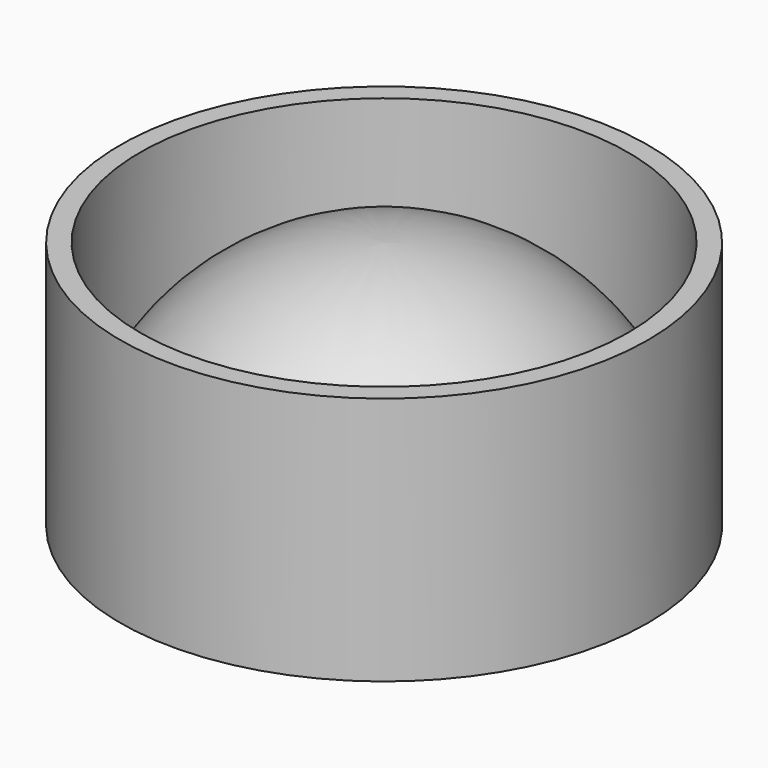
from build123d import *

# Parameters (mm, degrees)
F0_R     = 25
F1_DEPTH = 25
F2_R     = 24.99999
F3_R     = 26.5
F3_R_2   = 24.5
F4_DEPTH = 25


# Not quite as in the source:
# - a fillet or chamfer is up to 0.001 mm smaller than in the source, because OpenCascade refuses the exact size


with BuildPart() as f1:
    # F0 (on Top) → F1 (new body)
    with BuildSketch(Plane.XY):
        with Locations((-7.374277804, 10.7427751645)):
            Circle(F0_R)
    extrude(amount=F1_DEPTH)

    # F2 (radius 25 in the source; OpenCascade refuses exactly that, so slightly less here)
    f2_edges = [f1.edges().sort_by_distance(p)[0] for p in [
        (-32.374278, 10.742775, 25),
    ]]
    fillet(f2_edges, radius=F2_R)

    # F3 (on Top) → F4 (join)
    with BuildSketch(Plane.XY):
        with Locations((-7.374277804, 10.7427751645)):
            Circle(F3_R)
        with Locations((-7.374277804, 10.7427751645)):
            Circle(F3_R_2, mode=Mode.SUBTRACT)
    extrude(amount=F4_DEPTH)


solid = f1.part
